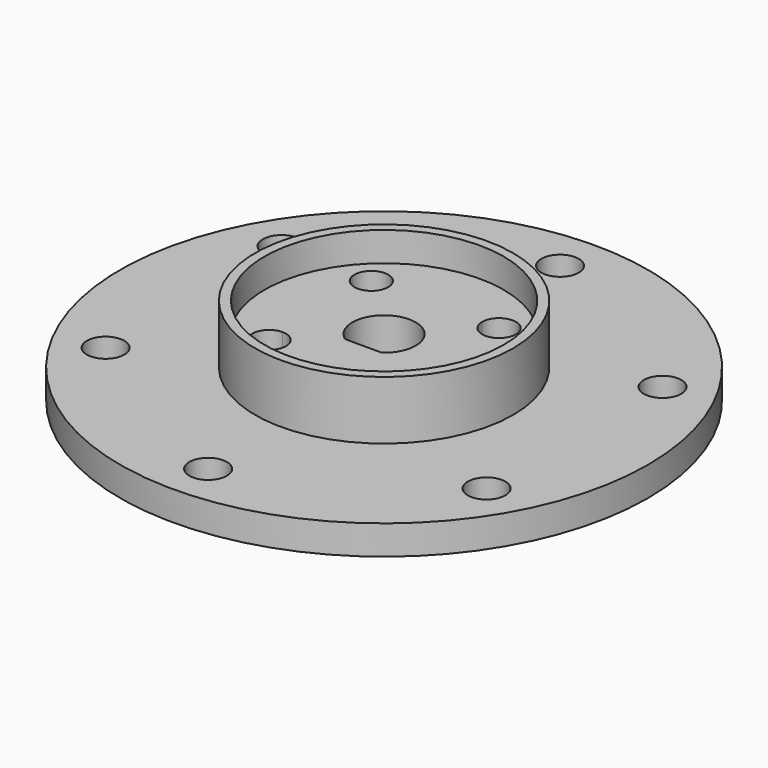
from build123d import *

# Parameters (mm, degrees)
F0_R     = 28.575
F0_R_2   = 2.032
F1_DEPTH = 3.175
F2_R     = 13.97
F3_DEPTH = 6.35
F5_DEPTH = 9.525
F7_DEPTH = 9.525
F8_R     = 12.954
F8_R_2   = 1.8288
F9_DEPTH = 3.175


with BuildPart() as f1:
    # F0 (on Top) → F1 (new body)
    with BuildSketch(Plane.XY):
        Circle(F0_R)
        with Locations((-20.6222299276, -11.90625)):
            Circle(F0_R_2, mode=Mode.SUBTRACT)
        with Locations((0, -23.8125)):
            Circle(F0_R_2, mode=Mode.SUBTRACT)
        with Locations((20.6222299276, -11.90625)):
            Circle(F0_R_2, mode=Mode.SUBTRACT)
        with Locations((-20.6222299276, 11.90625)):
            Circle(F0_R_2, mode=Mode.SUBTRACT)
        with Locations((20.6222299276, 11.90625)):
            Circle(F0_R_2, mode=Mode.SUBTRACT)
        with Locations((0, 23.8125)):
            Circle(F0_R_2, mode=Mode.SUBTRACT)
    extrude(amount=F1_DEPTH)

    # F2 (on face) → F3 (join)
    with BuildSketch(Plane.XY.offset(3.175)):
        Circle(F2_R)
    extrude(amount=F3_DEPTH)

    # F4 (on face) → F5 (cut, through all)
    with BuildSketch(Plane(origin=(0, 0, 0), x_dir=(1, 0, 0), z_dir=(0, 0, -1))):
        with BuildLine():
            ThreePointArc((-1.987864432, 2.794), (-1.5718864244, -3.0474930793), (3.429, 0))
            ThreePointArc((3.429, 0), (3.0474930793, 1.5718864244), (1.987864432, 2.794))
            Line((1.987864432, 2.794), (0, 2.794))
            Line((0, 2.794), (-1.987864432, 2.794))
        make_face()
    extrude(amount=-F5_DEPTH, mode=Mode.SUBTRACT)

    # F6 (on face) → F7 (cut, through all)
    with BuildSketch(Plane(origin=(0, 0, 0), x_dir=(1, 0, 0), z_dir=(0, 0, -1))):
        with BuildLine():
            Line((-6.9147972132, -6.9147972132), (-5.0859972132, -6.9147972132))
            ThreePointArc((-5.0859972132, -6.9147972132), (-5.6216403318, -5.6216403318), (-6.9147972132, -5.0859972132))
            Line((-6.9147972132, -5.0859972132), (-6.9147972132, -6.9147972132))
        make_face()
        with BuildLine():
            ThreePointArc((-6.9147972132, -5.0859972132), (-8.2079540947, -8.2079540947), (-5.0859972132, -6.9147972132))
            Line((-5.0859972132, -6.9147972132), (-6.9147972132, -6.9147972132))
            Line((-6.9147972132, -6.9147972132), (-6.9147972132, -5.0859972132))
        make_face()
        with BuildLine():
            Line((-6.9147972132, 6.9147972132), (-6.9147972132, 5.0859972132))
            ThreePointArc((-6.9147972132, 5.0859972132), (-5.6216403318, 5.6216403318), (-5.0859972132, 6.9147972132))
            Line((-5.0859972132, 6.9147972132), (-6.9147972132, 6.9147972132))
        make_face()
        with BuildLine():
            ThreePointArc((-5.0859972132, 6.9147972132), (-8.2079540947, 8.2079540947), (-6.9147972132, 5.0859972132))
            Line((-6.9147972132, 5.0859972132), (-6.9147972132, 6.9147972132))
            Line((-6.9147972132, 6.9147972132), (-5.0859972132, 6.9147972132))
        make_face()
        with BuildLine():
            Line((6.9147972132, 6.9147972132), (6.9147972132, 5.0859972132))
            ThreePointArc((6.9147972132, 5.0859972132), (8.2079540947, 5.6216403318), (8.7435972132, 6.9147972132))
            ThreePointArc((8.7435972132, 6.9147972132), (6.9147972132, 8.7435972132), (5.0859972132, 6.9147972132))
            Line((5.0859972132, 6.9147972132), (6.9147972132, 6.9147972132))
        make_face()
        with BuildLine():
            ThreePointArc((5.0859972132, 6.9147972132), (5.6216403318, 5.6216403318), (6.9147972132, 5.0859972132))
            Line((6.9147972132, 5.0859972132), (6.9147972132, 6.9147972132))
            Line((6.9147972132, 6.9147972132), (5.0859972132, 6.9147972132))
        make_face()
        with BuildLine():
            ThreePointArc((6.9147972132, -5.0859972132), (5.6216403318, -5.6216403318), (5.0859972132, -6.9147972132))
            Line((5.0859972132, -6.9147972132), (6.9147972132, -6.9147972132))
            Line((6.9147972132, -6.9147972132), (6.9147972132, -5.0859972132))
        make_face()
        with BuildLine():
            Line((6.9147972132, -6.9147972132), (5.0859972132, -6.9147972132))
            ThreePointArc((5.0859972132, -6.9147972132), (6.9147972132, -8.7435972132), (8.7435972132, -6.9147972132))
            ThreePointArc((8.7435972132, -6.9147972132), (8.2079540947, -5.6216403318), (6.9147972132, -5.0859972132))
            Line((6.9147972132, -5.0859972132), (6.9147972132, -6.9147972132))
        make_face()
    extrude(amount=-F7_DEPTH, mode=Mode.SUBTRACT)

    # F8 (on face) → F9 (cut)
    with BuildSketch(Plane.XY.offset(9.525)):
        Circle(F8_R)
        with Locations((-6.9147972132, -6.9147972132)):
            Circle(F8_R_2, mode=Mode.SUBTRACT)
        with Locations((6.9147972132, -6.9147972132)):
            Circle(F8_R_2, mode=Mode.SUBTRACT)
        with BuildLine():
            ThreePointArc((-1.987864432, -2.794), (0, 3.429), (1.987864432, -2.794))
            Line((1.987864432, -2.794), (-1.987864432, -2.794))
        make_face(mode=Mode.SUBTRACT)
        with Locations((-6.9147972132, 6.9147972132)):
            Circle(F8_R_2, mode=Mode.SUBTRACT)
        with Locations((6.9147972132, 6.9147972132)):
            Circle(F8_R_2, mode=Mode.SUBTRACT)
    extrude(amount=-F9_DEPTH, mode=Mode.SUBTRACT)


solid = f1.part
